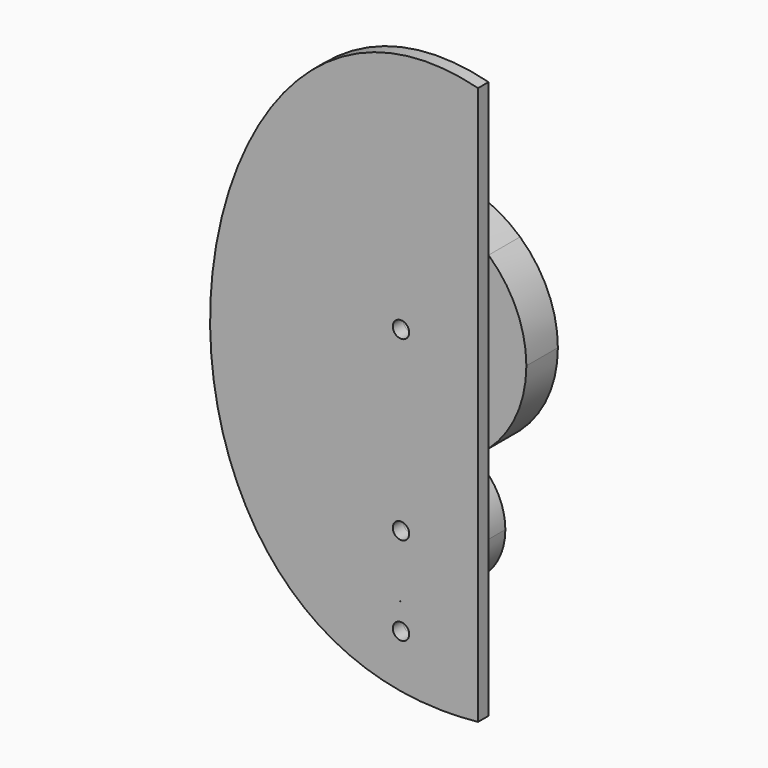
from build123d import *

# Parameters (mm, degrees)
F0_R     = 1.5875
F1_DEPTH = 2.54
F2_DEPTH = 7.62
F3_DEPTH = 7.62
F4_DEPTH = 7.62


# Not quite as in the source:
# - a feature names something its author has since deleted; it is built from what else it names


with BuildPart() as f1:
    # F0 (on Front) → F1 (new body)
    with BuildSketch(Plane.XZ):
        with BuildLine():
            Line((14.9111676306, 64.9484875902), (14.9111676306, 94.4228925787))
            add(Edge.make_bspline(
                [(14.9111676306, 94.4228925787), (-16.3680333644, 102.4050563574), (-54.9629772168, 39.3364652633), (-21.2016832001, -17.2942446428), (14.9111676306, -13.5271074213)],
                knots=[0, 0, 0, 0, 0.4983109993, 1, 1, 1, 1], degree=3))
            Line((14.9111676306, -13.5271074213), (14.9111676306, 31.9874375527))
            ThreePointArc((14.9111676306, 31.9874375527), (8.0811732468, 27.7642125741), (0.1961948099, 26.2438285592))
            ThreePointArc((0.1961948099, 26.2438285592), (8.6003289292, 22.6420175366), (12.065, 14.1804238741))
            ThreePointArc((12.065, 14.1804238741), (8.6571999537, 5.7770249212), (0.358889107, 2.1207628669))
            ThreePointArc((0.358889107, 2.1207628669), (3.7168236886, 0.516348123), (5.08, -2.9465439729))
            ThreePointArc((5.08, -2.9465439729), (-3.4628920959, -6.6633676615), (-0.358889107, 2.1207628669))
            ThreePointArc((-0.358889107, 2.1207628669), (-12.0647256139, 14.2617925558), (-0.1961948099, 26.2438285592))
            ThreePointArc((-0.1961948099, 26.2438285592), (-20.7037499974, 56.5491358183), (14.9111676306, 64.9484875902))
        make_face()
        with BuildLine():
            Line((14.9111676306, 31.9874375527), (14.9111676306, 64.9484875902))
            ThreePointArc((14.9111676306, 64.9484875902), (-20.7037499974, 56.5491358183), (-0.1961948099, 26.2438285592))
            ThreePointArc((-0.1961948099, 26.2438285592), (0, 26.2454238741), (0.1961948099, 26.2438285592))
            ThreePointArc((0.1961948099, 26.2438285592), (8.0811732468, 27.7642125741), (14.9111676306, 31.9874375527))
        make_face()
        with Locations((0, 48.4679625715)):
            Circle(F0_R, mode=Mode.SUBTRACT)
        with BuildLine():
            ThreePointArc((0.1961948099, 26.2438285592), (0, 26.2429625715), (-0.1961948099, 26.2438285592))
            ThreePointArc((-0.1961948099, 26.2438285592), (-12.0647256139, 14.2617925558), (-0.358889107, 2.1207628669))
            ThreePointArc((-0.358889107, 2.1207628669), (0, 2.1334560271), (0.358889107, 2.1207628669))
            ThreePointArc((0.358889107, 2.1207628669), (8.6571999537, 5.7770249212), (12.065, 14.1804238741))
            ThreePointArc((12.065, 14.1804238741), (8.6003289292, 22.6420175366), (0.1961948099, 26.2438285592))
        make_face()
        with Locations((0, 14.1804238741)):
            Circle(F0_R, mode=Mode.SUBTRACT)
        with BuildLine():
            ThreePointArc((0.358889107, 2.1207628669), (0, 2.1154238741), (-0.358889107, 2.1207628669))
            ThreePointArc((-0.358889107, 2.1207628669), (-3.4628920959, -6.6633676615), (5.08, -2.9465439729))
            ThreePointArc((5.08, -2.9465439729), (3.7168236886, 0.516348123), (0.358889107, 2.1207628669))
        make_face()
        with Locations((0, -2.9465439729)):
            Circle(F0_R, mode=Mode.SUBTRACT)
    extrude(amount=F1_DEPTH)


with BuildPart() as f2:
    # F0 (on Front) → F2 (new body)
    with BuildSketch(Plane.XZ):
        with BuildLine():
            Line((14.9111676306, 31.9874375527), (14.9111676306, 64.9484875902))
            ThreePointArc((14.9111676306, 64.9484875902), (-20.7037499974, 56.5491358183), (-0.1961948099, 26.2438285592))
            ThreePointArc((-0.1961948099, 26.2438285592), (0, 26.2454238741), (0.1961948099, 26.2438285592))
            ThreePointArc((0.1961948099, 26.2438285592), (8.0811732468, 27.7642125741), (14.9111676306, 31.9874375527))
        make_face()
        with Locations((0, 48.4679625715)):
            Circle(F0_R, mode=Mode.SUBTRACT)
        with BuildLine():
            ThreePointArc((22.225, 48.4679625715), (20.3144200703, 57.4832253078), (14.9111676306, 64.9484875902))
            Line((14.9111676306, 64.9484875902), (14.9111676306, 31.9874375527))
            ThreePointArc((14.9111676306, 31.9874375527), (20.3144200703, 39.4526998351), (22.225, 48.4679625715))
        make_face()
    extrude(amount=-F2_DEPTH)


with BuildPart() as f3:
    # F0 (on Front) → F3 (new body)
    with BuildSketch(Plane.XZ):
        with BuildLine():
            ThreePointArc((0.1961948099, 26.2438285592), (0, 26.2429625715), (-0.1961948099, 26.2438285592))
            ThreePointArc((-0.1961948099, 26.2438285592), (-12.0647256139, 14.2617925558), (-0.358889107, 2.1207628669))
            ThreePointArc((-0.358889107, 2.1207628669), (0, 2.1334560271), (0.358889107, 2.1207628669))
            ThreePointArc((0.358889107, 2.1207628669), (8.6571999537, 5.7770249212), (12.065, 14.1804238741))
            ThreePointArc((12.065, 14.1804238741), (8.6003289292, 22.6420175366), (0.1961948099, 26.2438285592))
        make_face()
        with Locations((0, 14.1804238741)):
            Circle(F0_R, mode=Mode.SUBTRACT)
    extrude(amount=-F3_DEPTH)


with BuildPart() as f4:
    # F0 (on Front) → F4 (new body)
    with BuildSketch(Plane.XZ):
        with BuildLine():
            ThreePointArc((0.358889107, 2.1207628669), (0, 2.1154238741), (-0.358889107, 2.1207628669))
            ThreePointArc((-0.358889107, 2.1207628669), (-3.4628920959, -6.6633676615), (5.08, -2.9465439729))
            ThreePointArc((5.08, -2.9465439729), (3.7168236886, 0.516348123), (0.358889107, 2.1207628669))
        make_face()
        with Locations((0, -2.9465439729)):
            Circle(F0_R, mode=Mode.SUBTRACT)
    extrude(amount=-F4_DEPTH)


solid = Compound([f1.part, f2.part, f3.part, f4.part])
